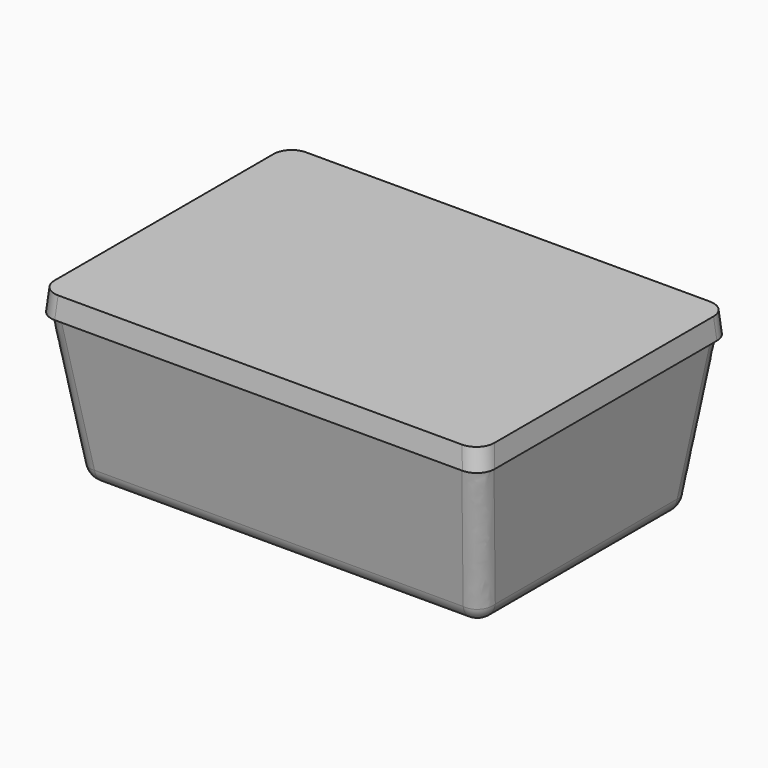
from build123d import *

# Parameters (mm, degrees)
F0_W        = 111.22
F0_H        = 71.63
F2_W        = 121.14
F2_H        = 85.07
F4_W        = 123.14
F4_H        = 87.07
F5_DEPTH    = 6
F6_T1_DEPTH = 118.265608958
F6_T3_DEPTH = 154.335608958
F9_R        = 5


# Not quite as in the source:
# - a fillet or chamfer that OpenCascade refuses, or shapes differently, is made with other operations: its cross-section is extruded or revolved along the edge and cut away or added
# - a feature of the source that left no trace in its solid (it failed there, or was rolled back) is left out


with BuildPart() as f3:
    # F0 (on Top) → F3 section 0
    with BuildSketch(Plane.XY):
        Rectangle(F0_W, F0_H)
    # F2 (on offset) → F3 section 1
    with BuildSketch(Plane.XY.offset(42)):
        Rectangle(F2_W, F2_H)
    loft()

    # F4 (on face) → F5 (join)
    with BuildSketch(Plane.XY.offset(42)):
        Rectangle(F4_W, F4_H)
    extrude(amount=F5_DEPTH)

    # F6: chamfer of 6 x 0.5249319812 on 4 edges, made by hand

    # F6_s2 → F6_t1 (cut)
    with BuildSketch(Plane.XZ.offset(-59.132804479)):
        Polygon((-61.57, 42), (-61.0450680188, 48), (-61.57, 48), align=None)
        Polygon((61.57, 42), (61.0450680188, 48), (61.57, 48), align=None)
    extrude(amount=F6_T1_DEPTH, mode=Mode.SUBTRACT)

    # F6_s4 → F6_t3 (cut)
    with BuildSketch(Plane.YZ.offset(-77.167804479)):
        Polygon((-43.0100680188, 48), (-43.535, 42), (-43.535, 48), align=None)
        Polygon((43.535, 42), (43.0100680188, 48), (43.535, 48), align=None)
    extrude(amount=F6_T3_DEPTH, mode=Mode.SUBTRACT)

    # F9
    f9_edges = [f3.edges().sort_by_distance(p)[0] for p in [
        (-61.307534, -43.272534, 45),
        (-61.307534, 43.272534, 45),
        (61.307534, 43.272534, 45),
        (61.307534, -43.272534, 45),
        (55.61, 0, 0),
        (58.09, 39.175, 21),
        (58.09, -39.175, 21),
        (0, 35.815, 0),
        (-58.09, 39.175, 21),
        (-55.61, 0, 0),
        (-58.09, -39.175, 21),
        (0, -35.815, 0),
    ]]
    fillet(f9_edges, radius=F9_R)


solid = f3.part
